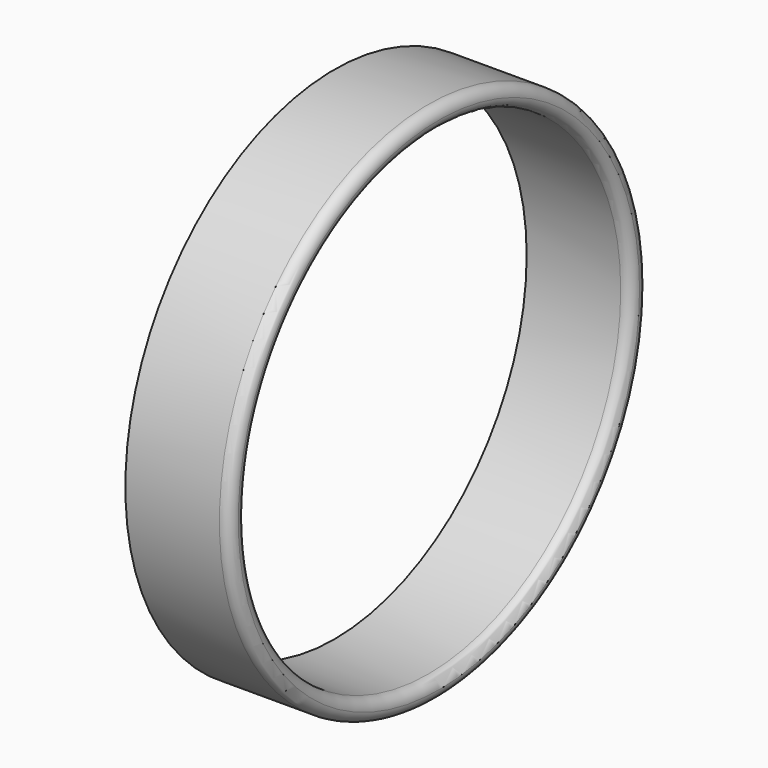
from build123d import *

# Parameters (mm, degrees)
F0_R     = 63.5
F0_R_2   = 58.42
F1_DEPTH = 25.4
F2_R     = 2.53999


# Not quite as in the source:
# - a fillet or chamfer is up to 0.001 mm smaller than in the source, because OpenCascade refuses the exact size


with BuildPart() as f1:
    # F0 (on Right) → F1 (new body)
    with BuildSketch(Plane.YZ):
        Circle(F0_R)
        Circle(F0_R_2, mode=Mode.SUBTRACT)
    extrude(amount=F1_DEPTH)

    # F2 (radius 2.54 in the source; OpenCascade refuses exactly that, so slightly less here)
    f2_edges = [f1.edges().sort_by_distance(p)[0] for p in [
        (25.4, -58.42, 0),
        (25.4, -63.5, 0),
    ]]
    fillet(f2_edges, radius=F2_R)


solid = f1.part
